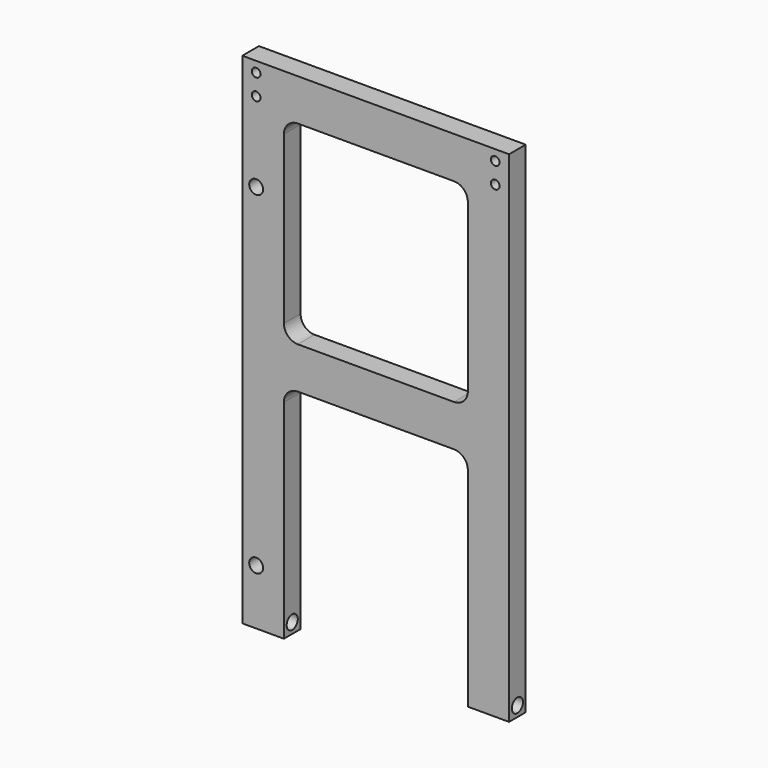
from build123d import *

# Parameters (mm, degrees)
F0_W     = 168.275
F0_H     = 177.8
F1_DEPTH = 9.525
F3_D     = 12.7
F5_D     = 12.7
F7_D     = 7.9375
F8_R     = 12.7


# Not quite as in the source:
# - a length typed as a fraction of an inch, garbled in the dataset ("3 / 203.2 mm" for 3/8 in), is restored


with BuildPart() as f1:
    # F0 (on Front) → F1 (new body, symmetric)
    with BuildSketch(Plane.XZ):
        Polygon((244.094, 0), (0, 0), (0, -457.2), (38.1, -457.2), (38.1, -254), (206.375, -254), (206.375, -457.2), (244.094, -457.2), align=None)
        with Locations((122.2375, -127)):
            Rectangle(F0_W, F0_H, mode=Mode.SUBTRACT)
    extrude(amount=F1_DEPTH, both=True)

    # F3 (through all)
    with Locations(Plane.YZ.offset(244.094)):
        with Locations((0, -447.675)):
            Hole(F3_D / 2)

    # F5 (through all)
    with Locations(Plane.XZ.offset(9.525)):
        with Locations((12.7, -406.4), (12.7, -101.6)):
            Hole(F5_D / 2)

    # F7 (through all)
    with Locations(Plane.XZ.offset(9.525)):
        with Locations((12.7, -9.525), (12.7, -28.575), (231.394, -28.575), (231.394, -9.525)):
            Hole(F7_D / 2)

    # F8
    f8_edges = [f1.edges().sort_by_distance(p)[0] for p in [
        (38.1, 0, -38.1),
        (206.375, 0, -38.1),
        (206.375, 0, -215.9),
        (38.1, 0, -215.9),
        (206.375, 0, -254),
        (38.1, 0, -254),
    ]]
    fillet(f8_edges, radius=F8_R)


solid = f1.part
